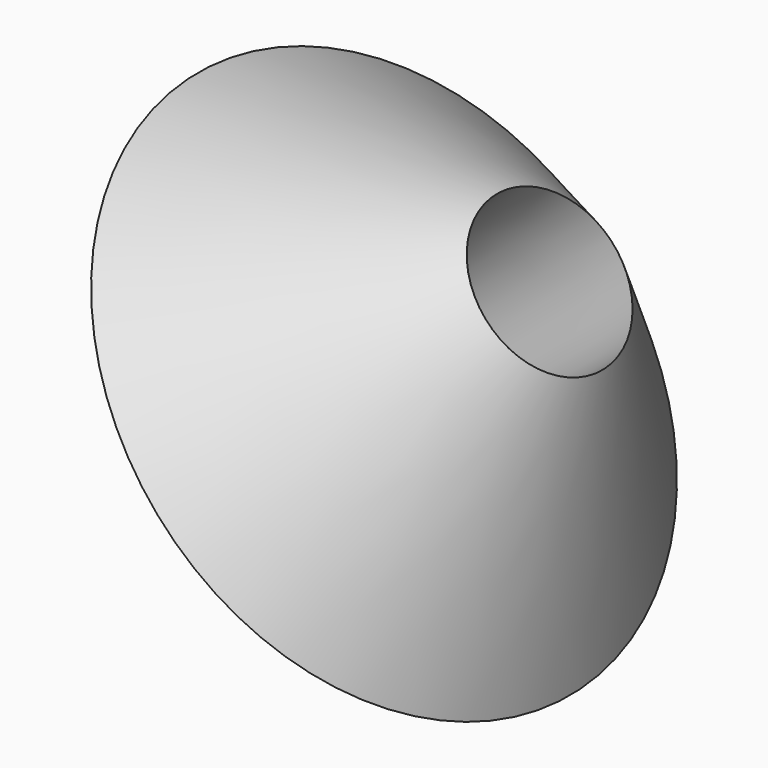
from build123d import *


with BuildPart() as f3:
    # F2 (on face) → F3 (revolve)
    with BuildSketch(Plane(origin=(-52.5687690169, 0, 60.5857061802), x_dir=(0.7553116107, 0, 0.6553658297), z_dir=(0.6553658297, 0, -0.7553116107))):
        Polygon((45.4506650567, 8.0647692084), (32.541668759, 20.0171601027), (19.4060392678, 7.3426626623), align=None)
    revolve(axis=Axis((-26.4949759178, -3.3436492085, 83.2093131865), (-0.7553116107, 0, -0.6553658297)))


solid = f3.part
